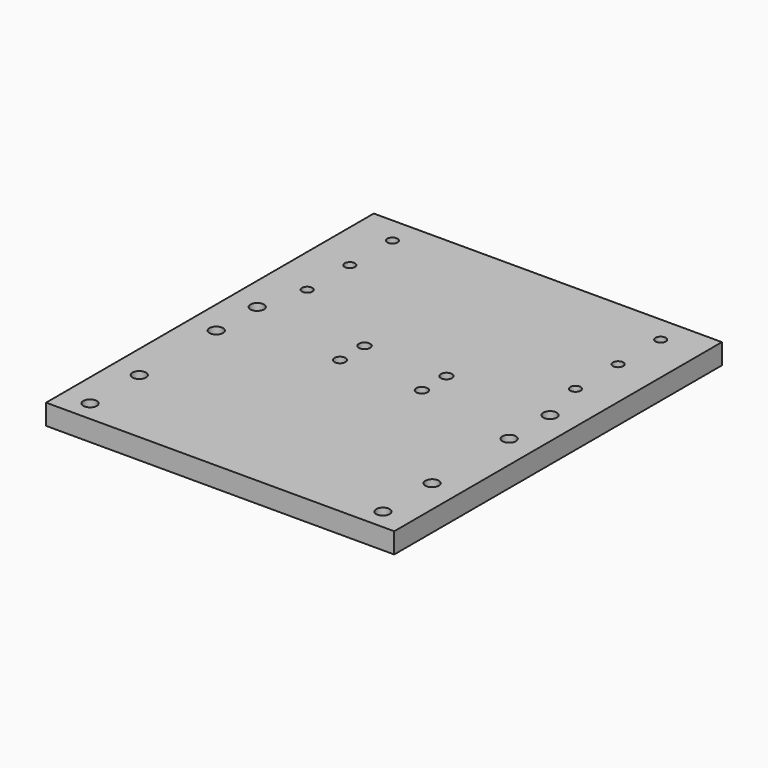
from build123d import *

# Parameters (mm, degrees)
F0_W           = 150
F0_H           = 200
F1_DEPTH       = 10
F3_D           = 5
F5_DEPTH       = 10
F6_DEPTH       = 10
F7_D           = 6.6
F7_CBORE_D     = 11.25
F7_CBORE_DEPTH = 6
F8_D           = 5.5
F8_CBORE_D     = 9.75
F8_CBORE_DEPTH = 5


# Not quite as in the source:
# - a feature names something its author has since deleted; it is built from what else it names


with BuildPart() as f1:
    # F0 (on Top) → F1 (new body)
    with BuildSketch(Plane.XY):
        with Locations((34.3934863061, 53.7353821645)):
            Rectangle(F0_W, F0_H)
    extrude(amount=F1_DEPTH)

    # F3 (through all)
    with Locations(Plane(origin=(0, 0, 0), x_dir=(1, 0, 0), z_dir=(0, 0, -1))):
        with Locations((-31.1065136939, -140.7353821645), (-31.1065136939, -114.7353821645), (-31.1065136939, -88.7353821645), (99.8934863061, -88.7353821645), (99.8934863061, -114.7353821645), (99.8934863061, -140.7353821645)):
            Hole(F3_D / 2)

    # F5 (add): a face of the model
    f5_faces = [f1.faces().sort_by_distance(p)[0] for p in [
        (109.3934863061, 53.7353821645, 5),
    ]]
    extrude(f5_faces, amount=F5_DEPTH)

    # F6 (add): a face of the model
    f6_faces = [f1.faces().sort_by_distance(p)[0] for p in [
        (-40.6065136939, 53.7353821645, 5),
    ]]
    extrude(f6_faces, amount=F6_DEPTH)

    # F7 (through all)
    with Locations(Plane(origin=(0, 0, 0), x_dir=(1, 0, 0), z_dir=(0, 0, -1))):
        with Locations((-37.1065136939, 36.2646178355), (-37.1065136939, 6.2646178355), (105.8934863061, 36.2646178355), (105.8934863061, 6.2646178355), (105.8934863061, -40.7353821645), (105.8934863061, -65.7353821645), (-37.1065136939, -65.7353821645), (-37.1065136939, -40.7353821645)):
            CounterBoreHole(F7_D / 2, F7_CBORE_D / 2, F7_CBORE_DEPTH)

    # F8 (through all)
    with Locations(Plane(origin=(0, 0, 0), x_dir=(1, 0, 0), z_dir=(0, 0, -1))):
        with Locations((54.8934863061, -51.2353821645), (54.8934863061, -66.2353821645), (14.8934863061, -51.2353821645), (14.8934863061, -66.2353821645)):
            CounterBoreHole(F8_D / 2, F8_CBORE_D / 2, F8_CBORE_DEPTH)


solid = f1.part
